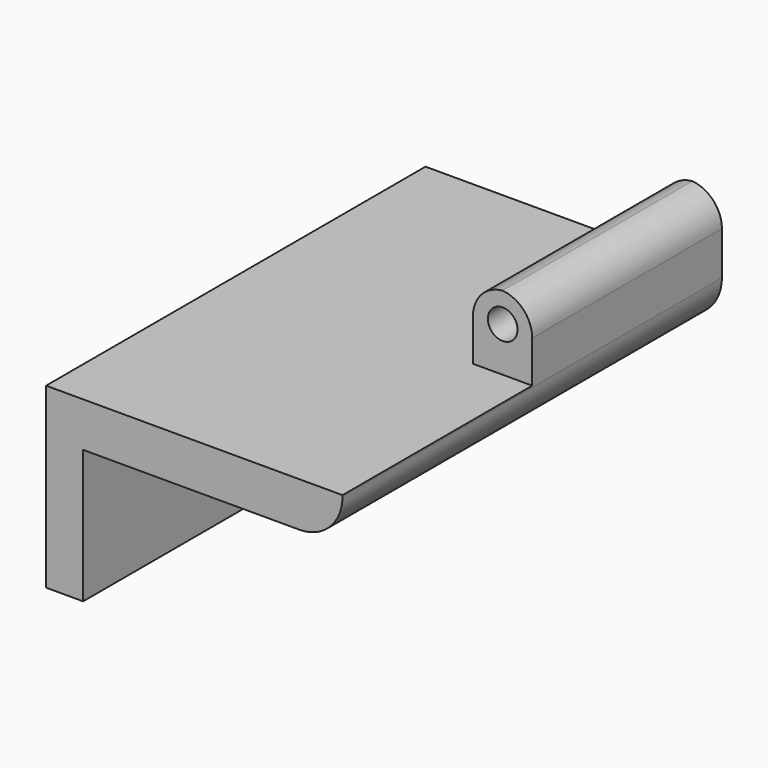
from build123d import *

# Parameters (mm, degrees)
F0_W        = 20
F0_H        = 32
F1_DEPTH    = 3
F2_W        = 2.5
F2_H        = 32
F3_DEPTH    = 9
F4_R        = 2.8970562748
F5_W        = 4
F5_H        = 16
F6_DEPTH    = 5
F7_R        = 1
F8_DEPTH    = 25
F9_T1_DEPTH = 26.8639610307


# Not quite as in the source:
# - a fillet or chamfer that OpenCascade refuses, or shapes differently, is made with other operations: its cross-section is extruded or revolved along the edge and cut away or added


with BuildPart() as f1:
    # F0 (on Top) → F1 (new body)
    with BuildSketch(Plane.XY):
        with Locations((-10, 0)):
            Rectangle(F0_W, F0_H)
    extrude(amount=F1_DEPTH)

    # F2 (on face) → F3 (join)
    with BuildSketch(Plane(origin=(0, 0, 0), x_dir=(1, 0, 0), z_dir=(0, 0, -1))):
        with Locations((-18.75, 0)):
            Rectangle(F2_W, F2_H)
    extrude(amount=F3_DEPTH)

    # F4
    f4_edges = [f1.edges().sort_by_distance(p)[0] for p in [
        (0, 0, 0),
    ]]
    fillet(f4_edges, radius=F4_R)

    # F5 (on face) → F6 (join)
    with BuildSketch(Plane.XY.offset(3)):
        with Locations((-2, 8)):
            Rectangle(F5_W, F5_H)
    extrude(amount=F6_DEPTH)

    # F7 (on face) → F8 (cut)
    with BuildSketch(Plane.XZ):
        with Locations((-1.9916295272, 5.9999883225)):
            Circle(F7_R)
    extrude(amount=-F8_DEPTH, mode=Mode.SUBTRACT)

    # F9: fillet of radius 2.1727922061 on 2 edges, made by hand

    # F9_s2 → F9_t1 (cut)
    with BuildSketch(Plane.XZ.offset(-21.4319805153)):
        with BuildLine():
            ThreePointArc((-1.8272077939, 8), (-3.3636038969, 7.3636038969), (-4, 5.8272077939))
            Line((-4, 5.8272077939), (-4, 8))
            Line((-4, 8), (-1.8272077939, 8))
        make_face()
        with BuildLine():
            ThreePointArc((0, 5.8272077939), (-0.6363961031, 7.3636038969), (-2.1727922061, 8))
            Line((-2.1727922061, 8), (0, 8))
            Line((0, 8), (0, 5.8272077939))
        make_face()
    extrude(amount=F9_T1_DEPTH, mode=Mode.SUBTRACT)


solid = f1.part
